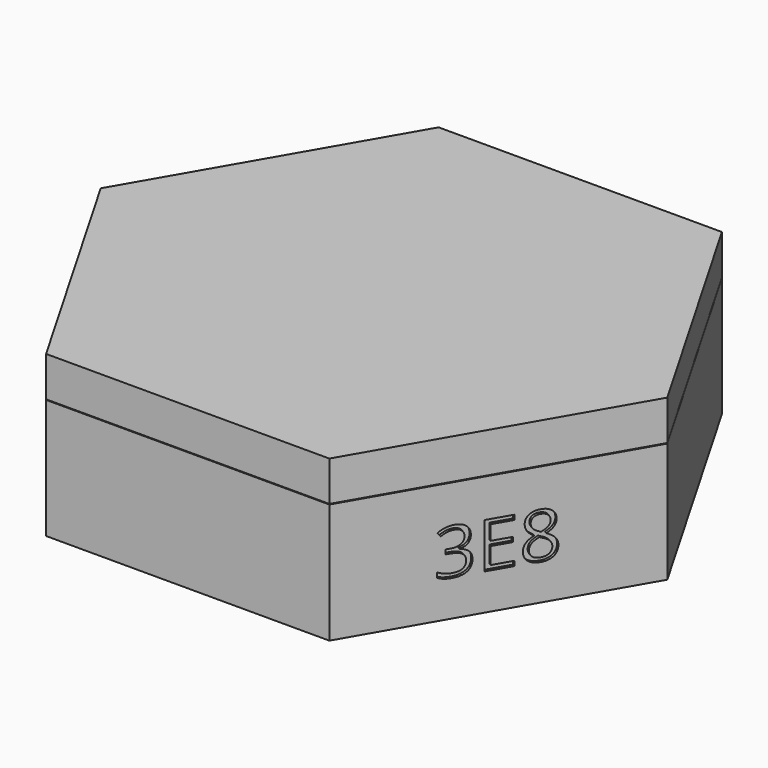
from build123d import *

# Parameters (mm, degrees)
F1_DEPTH     = 2
F3_DEPTH     = 24
F5_DEPTH     = 5
F6_TEXT_SIZE = 11.1241695575
F7_DEPTH     = 0.5
F8_R         = 12.6
F9_DEPTH     = 2.0010001
F12_DEPTH    = 2
F14_DEPTH    = 5


# Not quite as in the source:
# - Text() gives the source's letters only with a copy of the font that has no kerning and outlines rounded to 1/6400 em; it was checked with that copy


with BuildPart() as f1:
    # F0 (on Top) → F1 (new body)
    with BuildSketch(Plane.XY):
        Polygon((-24.8260615752, -43), (24.8260615752, -43), (49.6521231503, 0), (24.8260615752, 43), (-24.8260615752, 43), (-49.6521231503, 0), align=None)
    extrude(amount=F1_DEPTH)

    # F2 (on face) → F3 (join)
    with BuildSketch(Plane.XY.offset(2)):
        Polygon((-49.6521231503, 0), (-24.8260615752, -43), (24.8260615752, -43), (49.6521231503, 0), (24.8260615752, 43), (-24.8260615752, 43), align=None)
        Polygon((-23.6713610368, 41), (23.6713610368, 41), (47.3427220735, 0), (23.6713610368, -41), (-23.6713610368, -41), (-47.3427220735, 0), align=None, mode=Mode.SUBTRACT)
    extrude(amount=F3_DEPTH)

    # F4 (on face) → F5 (cut)
    with BuildSketch(Plane.XY.offset(26)):
        Polygon((-24.8260615752, 43), (-49.6521231503, 0), (-24.8260615752, -43), (24.8260615752, -43), (49.6521231503, 0), (24.8260615752, 43), align=None)
        Polygon((-24.0755062252, -41.7), (-48.1510124504, 0), (-24.0755062252, 41.7), (24.0755062252, 41.7), (48.1510124504, 0), (24.0755062252, -41.7), align=None, mode=Mode.SUBTRACT)
    extrude(amount=-F5_DEPTH, mode=Mode.SUBTRACT)

    # F6 (on face) → F7 (cut)
    with BuildSketch(Plane(origin=(37.2390923627, -21.5, 0), x_dir=(0.5, 0.8660254038, 0), z_dir=(0.8660254038, -0.5, 0))):
        with Locations((-9.5029046625, 6.3525000587)):
            Text('3E8', F6_TEXT_SIZE, font='Open Sans', text_align=(TextAlign.LEFT, TextAlign.BOTTOM))
    extrude(amount=-F7_DEPTH, mode=Mode.SUBTRACT)

    # F8 (on face) → F9 (cut, through all)
    with BuildSketch(Plane.XY.offset(2)):
        Circle(F8_R)
    extrude(amount=-F9_DEPTH, mode=Mode.SUBTRACT)


with BuildPart() as f12:
    # F11 (on offset) → F12 (new body)
    with BuildSketch(Plane.XY.offset(26.1)):
        Polygon((-24.8260615752, -43), (24.8260615752, -43), (49.6521231503, 0), (24.8260615752, 43), (-24.8260615752, 43), (-49.6521231503, 0), align=None)
    extrude(amount=F12_DEPTH)

    # F13 (on face) → F14 (join)
    with BuildSketch(Plane(origin=(0, 0, 26.1), x_dir=(1, 0, 0), z_dir=(0, 0, -1))):
        Polygon((49.6521231503, 0), (24.8260615752, 43), (-24.8260615752, 43), (-49.6521231503, 0), (-24.8260615752, -43), (24.8260615752, -43), align=None)
        Polygon((-24.4219163867, 42.3), (24.4219163867, 42.3), (48.8438327734, 0), (24.4219163867, -42.3), (-24.4219163867, -42.3), (-48.8438327734, 0), align=None, mode=Mode.SUBTRACT)
    extrude(amount=F14_DEPTH)


solid = Compound([f1.part, f12.part])
